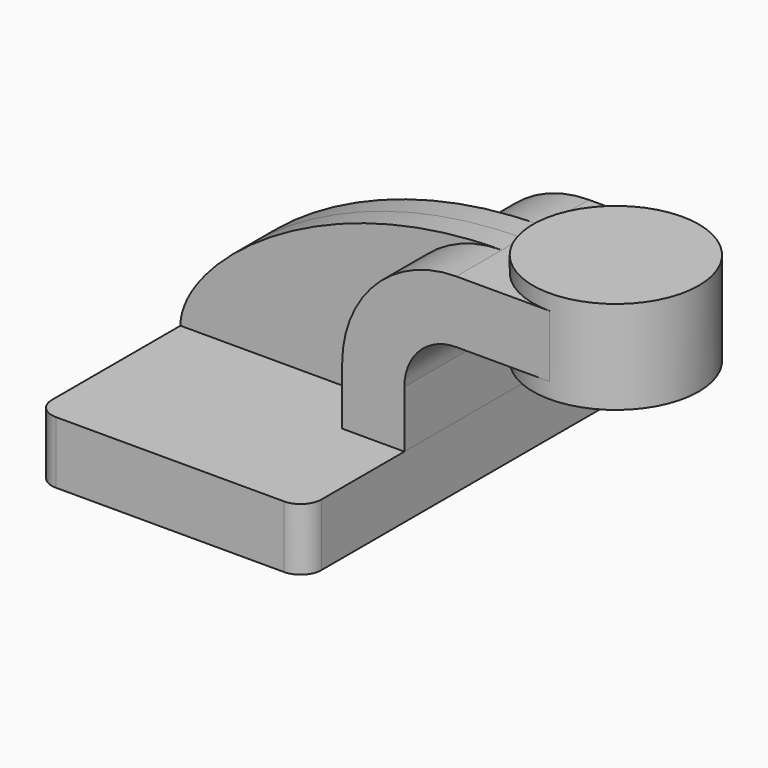
from build123d import *

# Parameters (mm, degrees)
F1_DEPTH = 63.5
F0_W     = 25.4
F0_H     = 19.05
F2_DEPTH = 25.4
F3_DEPTH = 7.9375
F5_R     = 6.35


with BuildPart() as f1:
    # F0 (on Front) → F1 (new body, symmetric)
    with BuildSketch(Plane.XZ):
        Polygon((41.275, -9.525), (41.275, 9.525), (22.225, 9.525), (-41.275, 9.525), (-41.275, -9.525), align=None)
    extrude(amount=F1_DEPTH, both=True)

    # F0 (on Front) → F3 (join, symmetric)
    with BuildSketch(Plane.XZ):
        with BuildLine():
            Line((-41.275, 9.525), (22.225, 9.525))
            Line((22.225, 9.525), (22.225, 27.0002))
            ThreePointArc((22.225, 27.0002), (32.4542956671, 51.6959043329), (57.15, 61.9252))
            add(Edge.make_bspline(
                [(-41.275, 9.525), (-41.275, 27.5978259742), (0, 61.9252), (57.15, 61.9252)],
                knots=[0, 0, 0, 0, 111.5045361635, 111.5045361635, 111.5045361635, 111.5045361635], degree=3))
        make_face()
    extrude(amount=F3_DEPTH, both=True)

    # F5
    f5_edges = [f1.edges().sort_by_distance(p)[0] for p in [
        (41.275, -63.5, 0),
        (-41.275, -63.5, 0),
        (41.275, 63.5, 0),
        (-41.275, 63.5, 0),
    ]]
    fillet(f5_edges, radius=F5_R)


with BuildPart() as f2:
    # F0 (on Front) → F2 (new body, symmetric)
    with BuildSketch(Plane.XZ):
        with BuildLine():
            Line((22.225, 9.525), (41.275, 9.525))
            Line((41.275, 9.525), (41.275, 27.0002))
            ThreePointArc((41.275, 27.0002), (45.9246798487, 38.2255201513), (57.15, 42.8752))
            Line((57.15, 42.8752), (60.325, 42.8752))
            Line((60.325, 42.8752), (60.325, 61.9252))
            Line((60.325, 61.9252), (57.15, 61.9252))
            ThreePointArc((57.15, 61.9252), (32.4542956671, 51.6959043329), (22.225, 27.0002))
            Line((22.225, 27.0002), (22.225, 9.525))
        make_face()
        with Locations((73.025, 52.4002)):
            Rectangle(F0_W, F0_H)
    extrude(amount=F2_DEPTH, both=True)

    # F0 (on Front) → F4 (revolve)
    with BuildSketch(Plane.XZ):
        Polygon((85.725, 61.9252), (85.725, 42.8752), (85.725, 38.1), (111.125, 38.1), (111.125, 66.675), (85.725, 66.675), align=None)
    revolve(axis=Axis((85.725, 0, 52.3875), (0, 0, 1)))


solid = Compound([f1.part, f2.part])
